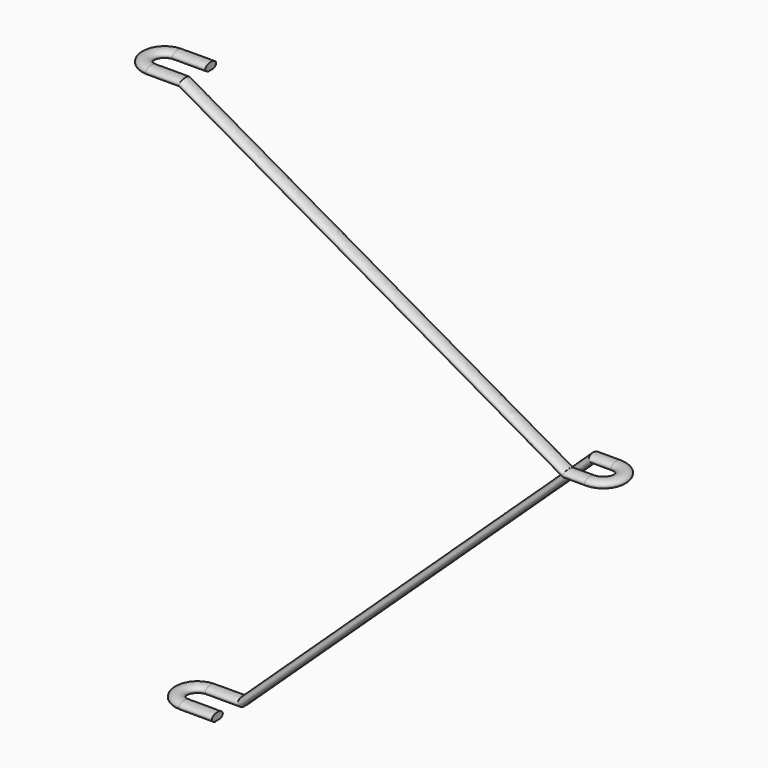
from build123d import *


# Not quite as in the source:
# - ends of sketch curves that miss each other by under 0.0002 mm in the source are joined


with BuildPart() as f15:
    # F15: sweep along a path in F8, F9, F7, F12, F11
    with BuildLine(Plane.XY.offset(1100)) as f15_path:
        Line((-1200, -150), (-1500, -150))
        ThreePointArc((-1500, -150), (-1650, 0), (-1500, 150))
        Line((-1500, 150), (-1200, 150))
    with BuildLine(Plane.XZ.offset(-150)) as f15_path_2:
        Line((-1200, 1100), (2000, 4100))
    with BuildLine(Plane.XY.offset(4100)) as f15_path_3:
        Line((2000, 150), (2200, 150))
        ThreePointArc((2200, 150), (2350, 0), (2200, -150))
        Line((2200, -150), (2000, -150))
    with BuildLine(Plane.XZ.offset(150)) as f15_path_4:
        Line((-1500, 6100), (2000, 4100))
    with BuildLine(Plane.XY.offset(6100)) as f15_path_5:
        Line((-1500, -150), (-1800, -150))
        ThreePointArc((-1800, -150), (-1950, 0), (-1800, 150))
        Line((-1800, 150), (-1500, 150))
    # F14 (on offset) → F15 (sweep)
    with BuildSketch(Plane.YZ.offset(-1350)):
        with BuildLine():
            Line((-129.75, 1070.0000286102), (-129.75, 1066.8880021744))
            add(Edge.make_bspline(
                [(-129.75, 1066.8880021744), (-49.2611179432, 1082.32460009), (-99.6305589716, 1120.7212819856), (-150, 1159.1179638813), (-200.3694410284, 1120.7212819856), (-250.7388820568, 1082.32460009), (-170.25, 1066.8880021744)],
                knots=[5.0423434982, 5.0423434982, 5.0423434982, 6.9167689221, 6.9167689221, 8.7911943459, 8.7911943459, 10.6656197697, 10.6656197697, 10.6656197697], degree=2, weights=[1, 0.5920366282, 1, 0.5920366282, 1, 0.5920366282, 1]))
            Line((-170.25, 1066.8880021744), (-170.25, 1070))
            Line((-170.25, 1070), (-150, 1070))
            Line((-150, 1070), (-129.75, 1070.0000286102))
        make_face()
    sweep(path=f15_path.line + f15_path_2.line + f15_path_3.line + f15_path_4.line + f15_path_5.line, transition=Transition.RIGHT)


solid = f15.part
